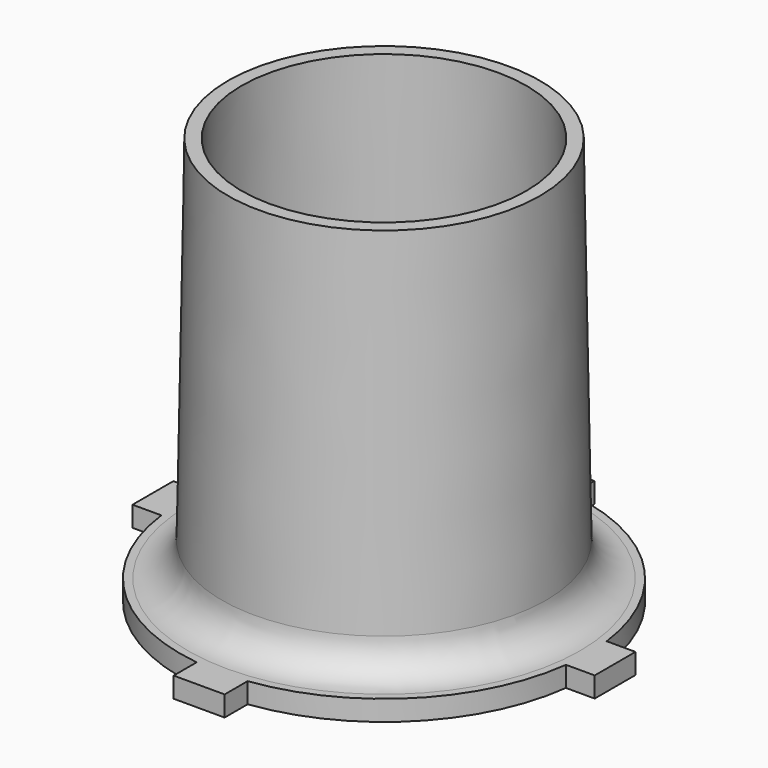
from build123d import *

# Parameters (mm, degrees)
F2_W            = 7.5
F2_H            = 8
F3_DEPTH        = 3
F3_COPIES_COUNT = 4
F4_R            = 5


# Not quite as in the source:
# - a pattern or mirror of a feature is missing from the dataset's text; its kind, count and spacing are read off the source's solid


with BuildPart() as f1:
    # F0 (on Front) → F1 (revolve)
    with BuildSketch(Plane.XZ):
        Polygon((23.9476348052, 3), (24, 0), (30, 0), (30, 3), align=None)
        Polygon((20.9525509577, 59.9908617094), (21.9473301491, 3), (23.9476348052, 3), (22.9528556138, 59.9908617094), align=None)
        Polygon((21.9473301491, 3), (21.9996953439, 0), (24, 0), (23.9476348052, 3), align=None)
    revolve(axis=Axis((0, 0, 53.7638920359), (0, 0, -1)))

    # F2 (on face) → F3 (join)
    with BuildSketch(Plane(origin=(0, 0, 0), x_dir=(1, 0, 0), z_dir=(0, 0, -1))):
        with Locations((0, 30)):
            Rectangle(F2_W, F2_H)
    f3 = extrude(amount=-F3_DEPTH)

    # F3_copies: F3 ×4 about axis
    f3_copies_axis = Axis((0, 0, 0), (0, 0, 1))
    for i in range(1, F3_COPIES_COUNT):
        add(f3.rotate(f3_copies_axis, i * 360 / F3_COPIES_COUNT))

    # F4
    f4_edges = [f1.edges().sort_by_distance(p)[0] for p in [
        (-23.947635, 0, 3),
        (-21.999695, 0, 0),
    ]]
    fillet(f4_edges, radius=F4_R)


solid = f1.part
